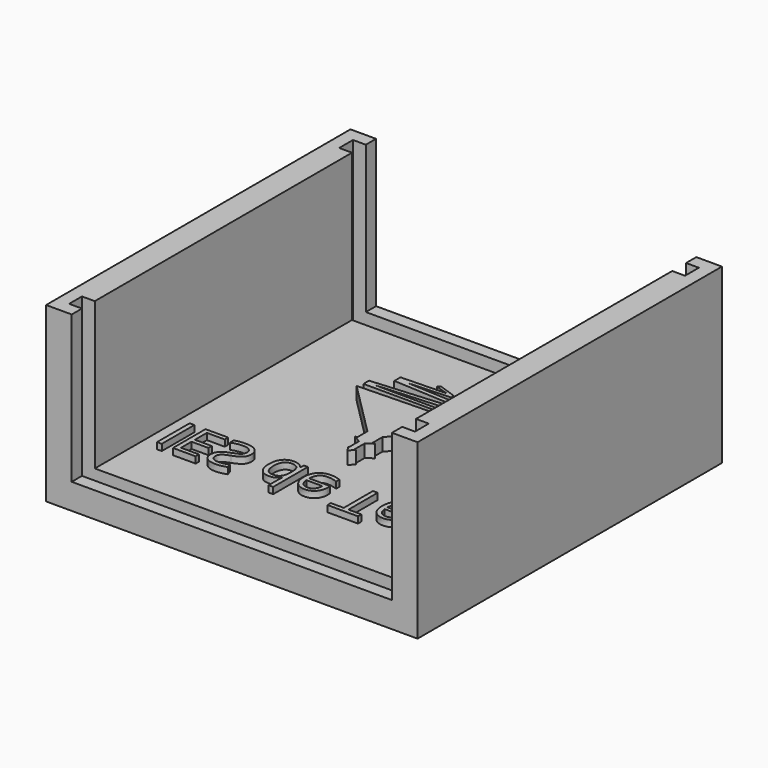
from build123d import *

# Parameters (mm, degrees)
F1_DEPTH     = 59.4
F3_DEPTH     = 25
F6_TEXT_SIZE = 8.9057558507
F7_DEPTH     = 3
F8_W         = 0.8984375745
F8_H         = 1.9921846688
F9_DEPTH     = 4
F10_W        = 54
F10_H        = 2.7
F11_DEPTH    = 25


# Not quite as in the source:
# - a feature names something its author has since deleted; it is built from what else it names
# - Text() gives the source's letters only with a copy of the font that has no kerning and outlines rounded to 1/6400 em; it was checked with that copy


with BuildPart() as f1:
    # F0 (on Front) → F1 (new body)
    with BuildSketch(Plane.XZ):
        Polygon((0, 27), (0, 0), (58, 0), (58, 27), (54, 27), (54, 4), (4, 4), (4, 27), align=None)
    extrude(amount=F1_DEPTH)

    # F2 (on face) → F3 (cut)
    with BuildSketch(Plane.XY.offset(27)):
        Polygon((54, -54.7074074074), (2, -54.9), (2, -57.4), (54, -57.4), align=None)
        Polygon((56, -54.7), (54, -54.7074074074), (54, -57.4), (56, -57.4), align=None)
    extrude(amount=-F3_DEPTH, mode=Mode.SUBTRACT)

    # F6 (on offset) → F7 (join)
    with BuildSketch(Plane(origin=(0, 0, 2), x_dir=(1, 0, 0), z_dir=(0, 0, -1))):
        with Locations((5.8981006123, 39.8505934059)):
            Text('IES de Teis', F6_TEXT_SIZE, font='Open Sans', text_align=(TextAlign.LEFT, TextAlign.BOTTOM))
    extrude(amount=-F7_DEPTH)

    # F8 (on offset) → F9 (join)
    with BuildSketch(Plane(origin=(0, 0, 2), x_dir=(1, 0, 0), z_dir=(0, 0, -1))):
        Polygon((28.1812131841, 34.163199014), (27.4976205517, 34.963979966), (26.9898076046, 34.163199014), (27.0679325301, 34.163199014), (27.9663701046, 34.163199014), align=None)
        with Locations((27.5171513174, 33.1671066796)):
            Rectangle(F8_W, F8_H)
        Polygon((27.9663701046, 32.1710143452), (27.0679325301, 32.1710143452), (25.8374635566, 31.4483564561), (26.2280881841, 31.4483564561), (26.2280881841, 29.475699759), (28.6109012056, 29.475699759), (28.6109012056, 31.4678881531), (29.0015258331, 31.4678881531), align=None)
        Polygon((28.6109012056, 29.475699759), (26.2280881841, 29.475699759), (17.6929302949, 20.9210101729), (35.8179334987, 20.4131990885), (36.7554326046, 21.3506981944), align=None)
        Polygon((36.4535443921, 19.9894063388), (18.055106743, 19.9894063388), (18.0194110114, 19.4481533235), (18.055106743, 18.8956573819), (33.4189922925, 17.7087680147), (20.457345822, 17.0229088492), (20.476981296, 16.5128443604), (20.457345822, 15.8120069035), (27.5472663167, 15.6133674785), (25.4569606755, 14.9695179735), (25.8285452116, 14.5987818231), (28.6109012056, 15.5835674514), (28.5905295184, 16.1127563185), (22.0689556139, 16.434342345), (34.8454470071, 17.0659737017), (35.3388032839, 17.5604589658), (35.3597954351, 18.3097195094), (19.1819940886, 19.3718272251), (36.981378371, 19.4627774876), align=None)
    extrude(amount=-F9_DEPTH)

    # F10 (on face) → F11 (cut)
    with BuildSketch(Plane.XY.offset(27)):
        with Locations((29, -3.35)):
            Rectangle(F10_W, F10_H)
    extrude(amount=-F11_DEPTH, mode=Mode.SUBTRACT)


solid = f1.part
